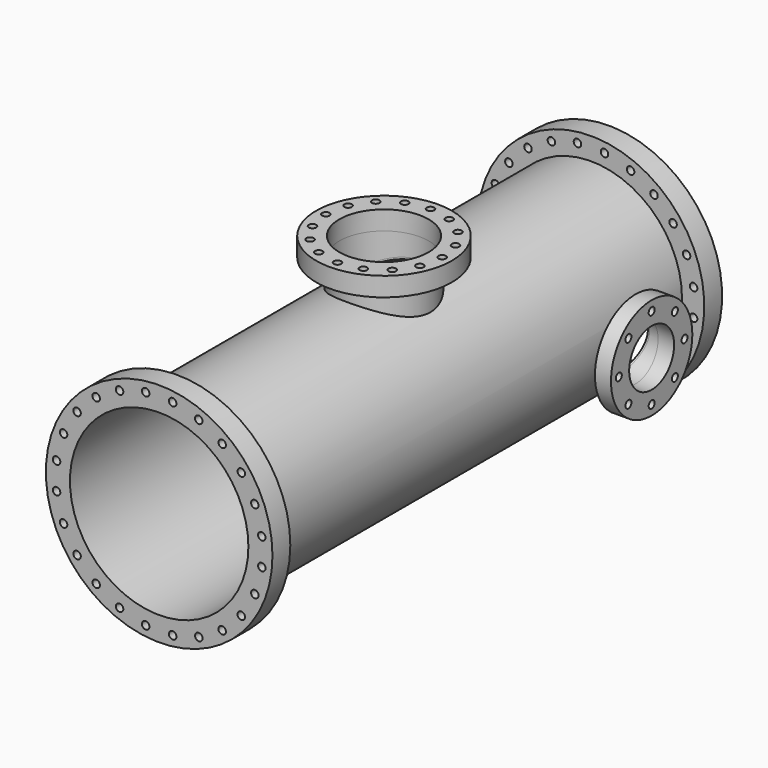
from build123d import *

# Parameters (mm, degrees)
F0_R      = 102
F0_R_2    = 100
F1_DEPTH  = 580
F2_R      = 127
F2_R_2    = 102
F2_R_3    = 100
F3_DEPTH  = 25
F4_R      = 127
F4_R_2    = 102
F4_R_3    = 100
F5_DEPTH  = 25
F7_D      = 8.4
F9_R      = 52
F9_R_2    = 50
F10_REACH = 399.0792104868
F11_REACH = 393.4223562373
F9_R_3    = 76
F12_DEPTH = 21.3
F14_D     = 8.4
F14_DEPTH = 27
F14_TIP   = 2.5236145999
F16_R     = 33.5
F16_R_2   = 31.5
F17_REACH = 331.753308679
F18_REACH = 326.0964544295
F16_R_3   = 57
F19_DEPTH = 18
F21_D     = 8.4
F21_DEPTH = 24
F21_TIP   = 2.5236145999


with BuildPart() as f1:
    # F0 (on Front) → F1 (new body)
    with BuildSketch(Plane.XZ):
        Circle(F0_R)
        Circle(F0_R_2, mode=Mode.SUBTRACT)
    extrude(amount=F1_DEPTH)

    # F2 (on face) → F3 (join)
    with BuildSketch(Plane.XZ.offset(580)):
        Circle(F2_R)
        Circle(F2_R_2, mode=Mode.SUBTRACT)
        Circle(F2_R_2)
        Circle(F2_R_3, mode=Mode.SUBTRACT)
    extrude(amount=F3_DEPTH)

    # F4 (on face) → F5 (join)
    with BuildSketch(Plane(origin=(0, 0, 0), x_dir=(-1, 0, 0), z_dir=(0, 1, 0))):
        Circle(F4_R)
        Circle(F4_R_2, mode=Mode.SUBTRACT)
        Circle(F4_R_2)
        Circle(F4_R_3, mode=Mode.SUBTRACT)
    extrude(amount=F5_DEPTH)

    # F7 (through all)
    with Locations(Plane(origin=(0, 25, 0), x_dir=(-1, 0, 0), z_dir=(0, 1, 0))):
        with Locations((15.1410382975, 115.0076039194), (44.3912781544, 107.1700257713), (70.616325765, 92.0289874738), (92.0289874738, 70.616325765), (107.1700257713, 44.3912781544), (115.0076039194, 15.1410382975), (115.0076039194, -15.1410382975), (107.1700257713, -44.3912781544), (92.0289874738, -70.616325765), (70.616325765, -92.0289874738), (44.3912781544, -107.1700257713), (15.1410382975, -115.0076039194), (-15.1410382975, -115.0076039194), (-44.3912781544, -107.1700257713), (-70.616325765, -92.0289874738), (-92.0289874738, -70.616325765), (-107.1700257713, -44.3912781544), (-115.0076039194, -15.1410382975), (-115.0076039194, 15.1410382975), (-107.1700257713, 44.3912781544), (-92.0289874738, 70.616325765), (-70.616325765, 92.0289874738), (-44.3912781544, 107.1700257713), (-15.1410382975, 115.0076039194)):
            Hole(F7_D / 2)

    f10_end = f1.faces().sort_by_distance((-102, -290, 0))[0]
    # F9 (on offset) → F10 (join, up to a face of the model that its end follows)
    with BuildSketch(Plane.XY.offset(125)):
        with Locations((0, -290)):
            Circle(F9_R)
        with Locations((0, -290)):
            Circle(F9_R_2, mode=Mode.SUBTRACT)
    f10_long = extrude(amount=-F10_REACH, mode=Mode.PRIVATE)
    add(split(f10_long, bisect_by=f10_end, keep=Keep.ALL, mode=Mode.PRIVATE).solids().sort_by_distance((-50.5292178951, -290, 125))[0])

    f11_end = f1.faces().sort_by_distance((-100, -302.5, 0))[0]
    # F9 (on offset) → F11 (cut, up to a face of the model that its end follows)
    with BuildSketch(Plane.XY.offset(125)):
        with Locations((0, -290)):
            Circle(F9_R_2)
    f11_long = extrude(amount=-F11_REACH, mode=Mode.PRIVATE)
    add(split(f11_long, bisect_by=f11_end, keep=Keep.ALL, mode=Mode.PRIVATE).solids().sort_by_distance((0, -290, 125))[0], mode=Mode.SUBTRACT)

    # F9 (on offset) → F12 (join)
    with BuildSketch(Plane.XY.offset(125)):
        with Locations((0, -290)):
            Circle(F9_R_3)
        with Locations((0, -290)):
            Circle(F9_R, mode=Mode.SUBTRACT)
        with Locations((0, -290)):
            Circle(F9_R)
        with Locations((0, -290)):
            Circle(F9_R_2, mode=Mode.SUBTRACT)
    extrude(amount=F12_DEPTH)

    # F14
    with Locations(Plane.XY.offset(146.3)):
        with Locations((0, -224.85), (24.9318256186, -229.8092484569), (46.0680067943, -243.9319932057), (60.1907515431, -265.0681743814), (65.15, -290), (60.1907515431, -314.9318256186), (46.0680067943, -336.0680067943), (24.9318256186, -350.1907515431), (0, -355.15), (-24.9318256186, -350.1907515431), (-46.0680067943, -336.0680067943), (-60.1907515431, -314.9318256186), (-65.15, -290), (-60.1907515431, -265.0681743814), (-46.0680067943, -243.9319932057), (-24.9318256186, -229.8092484569)):
            Hole(F14_D / 2, depth=F14_DEPTH)
            with Locations((0, 0, -(F14_DEPTH + F14_TIP / 2))):  # 118° drill point
                Cone(0, F14_D / 2, F14_TIP, mode=Mode.SUBTRACT)

    f17_end = f1.faces().sort_by_distance((-102, -290, 0))[0]
    # F16 (on offset) → F17 (join, up to a face of the model that its end follows)
    with BuildSketch(Plane.YZ.offset(110)):
        with Locations((-75, -20)):
            Circle(F16_R)
        with Locations((-75, -20)):
            Circle(F16_R_2, mode=Mode.SUBTRACT)
    f17_long = extrude(amount=-F17_REACH, mode=Mode.PRIVATE)
    add(split(f17_long, bisect_by=f17_end, keep=Keep.ALL, mode=Mode.PRIVATE).solids().sort_by_distance((110, -107.5524769132, -20))[0])

    f18_end = f1.faces().sort_by_distance((-100, -302.5, 0))[0]
    # F16 (on offset) → F18 (cut, up to a face of the model that its end follows)
    with BuildSketch(Plane.YZ.offset(110)):
        with Locations((-75, -20)):
            Circle(F16_R_2)
    f18_long = extrude(amount=-F18_REACH, mode=Mode.PRIVATE)
    add(split(f18_long, bisect_by=f18_end, keep=Keep.ALL, mode=Mode.PRIVATE).solids().sort_by_distance((110, -75, -20))[0], mode=Mode.SUBTRACT)

    # F16 (on offset) → F19 (join)
    with BuildSketch(Plane.YZ.offset(110)):
        with Locations((-75, -20)):
            Circle(F16_R_3)
        with Locations((-75, -20)):
            Circle(F16_R, mode=Mode.SUBTRACT)
        with Locations((-75, -20)):
            Circle(F16_R)
        with Locations((-75, -20)):
            Circle(F16_R_2, mode=Mode.SUBTRACT)
    extrude(amount=F19_DEPTH)

    # F21
    with Locations(Plane.YZ.offset(128)):
        with Locations((-75, 26), (-42.4730880654, 12.5269119346), (-29, -20), (-42.4730880654, -52.5269119346), (-75, -66), (-107.5269119346, -52.5269119346), (-121, -20), (-107.5269119346, 12.5269119346)):
            Hole(F21_D / 2, depth=F21_DEPTH)
            with Locations((0, 0, -(F21_DEPTH + F21_TIP / 2))):  # 118° drill point
                Cone(0, F21_D / 2, F21_TIP, mode=Mode.SUBTRACT)


solid = f1.part
